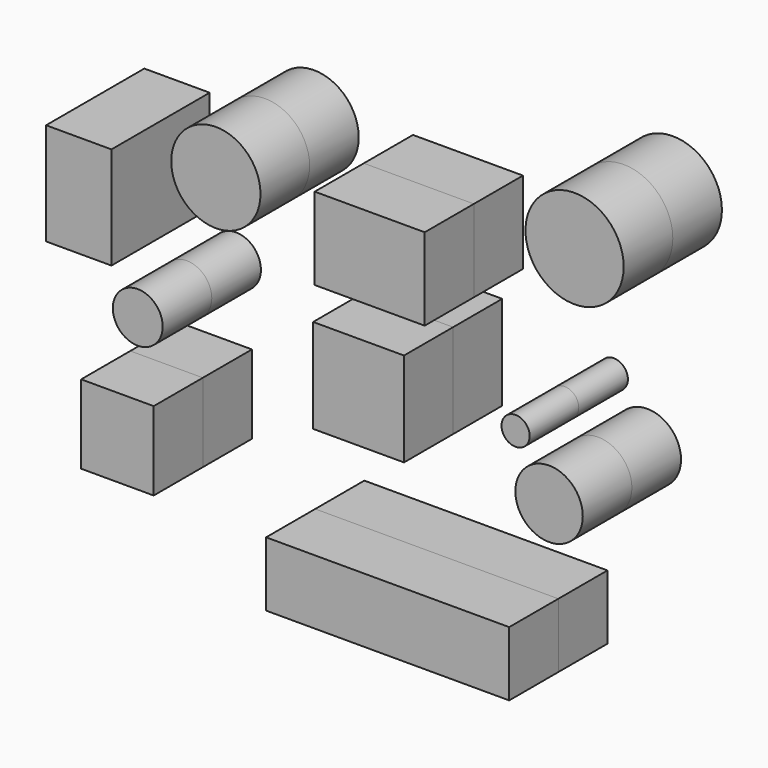
from build123d import *

# Parameters (mm, degrees)
F0_W     = 26.613753289
F0_H     = 41.6500791907
F1_DEPTH = 25
F0_W_2   = 44.7890106589
F0_H_2   = 33.482324332
F0_W_3   = 36.9996093214
F0_H_3   = 38.3273893967
F0_W_4   = 29.534779489
F0_H_4   = 32.0437960327
F0_W_5   = 98.9901963621
F0_H_5   = 26.2742973864
F0_R     = 18.1752443314
F0_R_2   = 10.148267962
F0_R_3   = 5.7257656008
F0_R_4   = 13.7270743948
F0_R_5   = 19.9959609748
F2_DEPTH = 25


with BuildPart() as f1:
    # F0 (on Front) → F1 (new body)
    with BuildSketch(Plane.XZ):
        with Locations((-68.3194566518, 56.8735636771)):
            Rectangle(F0_W, F0_H)
    extrude(amount=F1_DEPTH)

    # F2 (add): a face of the model
    f2_faces = [f1.faces().sort_by_distance(p)[0] for p in [
        (-68.3194566518, -25, 56.8735636771),
    ]]
    extrude(f2_faces, amount=F2_DEPTH)


with BuildPart() as f1b:
    # F0 (on Front) → F1, piece 2 (new body)
    with BuildSketch(Plane.XZ):
        with Locations((50.1442132518, 72.7335456759)):
            Rectangle(F0_W_2, F0_H_2)
    extrude(amount=F1_DEPTH)


with BuildPart() as f1c:
    # F0 (on Front) → F1, piece 3 (new body)
    with BuildSketch(Plane.XZ):
        with Locations((45.600393787, 23.3872788958)):
            Rectangle(F0_W_3, F0_H_3)
    extrude(amount=F1_DEPTH)


with BuildPart() as f1d:
    # F0 (on Front) → F1, piece 4 (new body)
    with BuildSketch(Plane.XZ):
        with Locations((-52.5783933699, -24.7525367886)):
            Rectangle(F0_W_4, F0_H_4)
    extrude(amount=F1_DEPTH)


with BuildPart() as f1e:
    # F0 (on Front) → F1, piece 5 (new body)
    with BuildSketch(Plane.XZ):
        with Locations((57.4467657134, -54.0079157799)):
            Rectangle(F0_W_5, F0_H_5)
    extrude(amount=F1_DEPTH)


with BuildPart() as f1f:
    # F0 (on Front) → F1, piece 6 (new body)
    with BuildSketch(Plane.XZ):
        with Locations((-12.4954786152, 81.4270600677)):
            Circle(F0_R)
    extrude(amount=F1_DEPTH)


with BuildPart() as f1g:
    # F0 (on Front) → F1, piece 7 (new body)
    with BuildSketch(Plane.XZ):
        with Locations((-44.3021655083, 20.9651011974)):
            Circle(F0_R_2)
    extrude(amount=F1_DEPTH)


with BuildPart() as f1h:
    # F0 (on Front) → F1, piece 8 (new body)
    with BuildSketch(Plane.XZ):
        with Locations((109.5383316278, 30.3227584809)):
            Circle(F0_R_3)
    extrude(amount=F1_DEPTH)


with BuildPart() as f1i:
    # F0 (on Front) → F1, piece 9 (new body)
    with BuildSketch(Plane.XZ):
        with Locations((123.1697648764, 8.6177336052)):
            Circle(F0_R_4)
    extrude(amount=F1_DEPTH)


with BuildPart() as f1j:
    # F0 (on Front) → F1, piece 10 (new body)
    with BuildSketch(Plane.XZ):
        with Locations((133.5556060076, 103.4657880664)):
            Circle(F0_R_5)
    extrude(amount=F1_DEPTH)


with BuildPart() as f2:
    # F2#2 (new): a face of the model
    f2_2_faces = [f1b.part.faces().sort_by_distance(p)[0] for p in [
        (50.1442132518, -25, 72.7335456759),
    ]]
    extrude(f2_2_faces, amount=F2_DEPTH)


with BuildPart() as f2b:
    # F2#3 (new): a face of the model
    f2_3_faces = [f1f.part.faces().sort_by_distance(p)[0] for p in [
        (-12.4954786152, -25, 81.4270600677),
    ]]
    extrude(f2_3_faces, amount=F2_DEPTH)


with BuildPart() as f2c:
    # F2#4 (new): a face of the model
    f2_4_faces = [f1g.part.faces().sort_by_distance(p)[0] for p in [
        (-44.3021655083, -25, 20.9651011974),
    ]]
    extrude(f2_4_faces, amount=F2_DEPTH)


with BuildPart() as f2d:
    # F2#5 (new): a face of the model
    f2_5_faces = [f1d.part.faces().sort_by_distance(p)[0] for p in [
        (-52.5783933699, -25, -24.7525367886),
    ]]
    extrude(f2_5_faces, amount=F2_DEPTH)


with BuildPart() as f2e:
    # F2#6 (new): a face of the model
    f2_6_faces = [f1e.part.faces().sort_by_distance(p)[0] for p in [
        (57.4467657134, -25, -54.0079157799),
    ]]
    extrude(f2_6_faces, amount=F2_DEPTH)


with BuildPart() as f2f:
    # F2#7 (new): a face of the model
    f2_7_faces = [f1i.part.faces().sort_by_distance(p)[0] for p in [
        (123.1697648764, -25, 8.6177336052),
    ]]
    extrude(f2_7_faces, amount=F2_DEPTH)


with BuildPart() as f2g:
    # F2#8 (new): a face of the model
    f2_8_faces = [f1c.part.faces().sort_by_distance(p)[0] for p in [
        (45.600393787, -25, 23.3872788958),
    ]]
    extrude(f2_8_faces, amount=F2_DEPTH)


with BuildPart() as f2h:
    # F2#9 (new): a face of the model
    f2_9_faces = [f1h.part.faces().sort_by_distance(p)[0] for p in [
        (109.5383316278, -25, 30.3227584809),
    ]]
    extrude(f2_9_faces, amount=F2_DEPTH)


with BuildPart() as f2i:
    # F2#10 (new): a face of the model
    f2_10_faces = [f1j.part.faces().sort_by_distance(p)[0] for p in [
        (133.5556060076, -25, 103.4657880664),
    ]]
    extrude(f2_10_faces, amount=F2_DEPTH)


solid = Compound([f1.part, f1b.part, f1c.part, f1d.part, f1e.part, f1f.part, f1g.part, f1h.part, f1i.part, f1j.part, f2.part, f2b.part, f2c.part, f2d.part, f2e.part, f2f.part, f2g.part, f2h.part, f2i.part])
